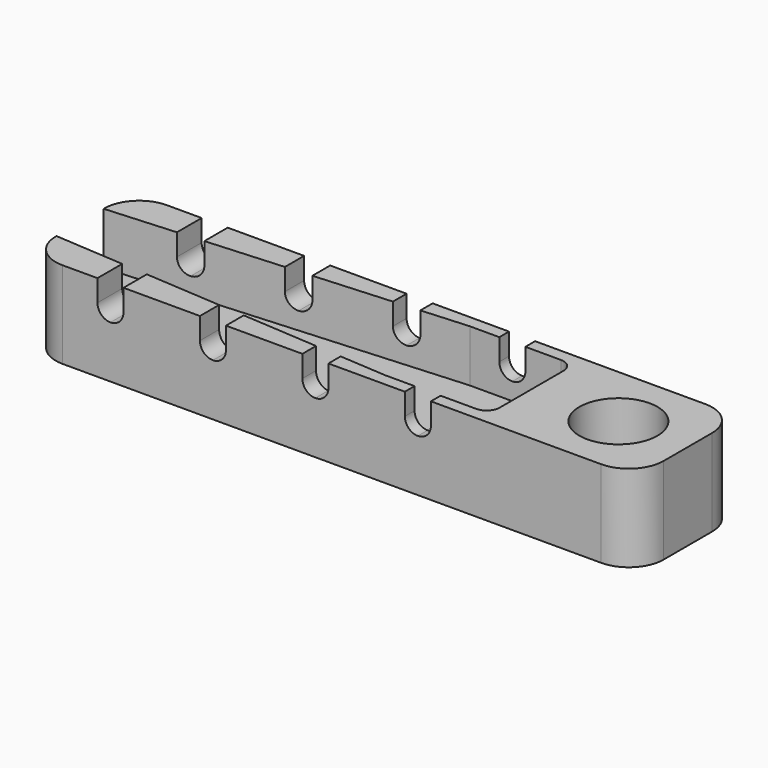
from build123d import *

# Parameters (mm, degrees)
F0_W     = 1.5
F0_H     = 0.7
F0_R     = 2.25
F0_H_2   = 6.1
F0_W_2   = 2.8
F1_DEPTH = 5
F2_DEPTH = 3
F3_DEPTH = 2
F4_R     = 0.74999
F5_R     = 2


# Not quite as in the source:
# - a fillet or chamfer is up to 0.001 mm smaller than in the source, because OpenCascade refuses the exact size


with BuildPart() as f1:
    # F0 (on Top) → F1 (new body)
    with BuildSketch(Plane.XY):
        Polygon((-18.8879279066, 3.75), (-22.8879279066, 3.75), (-22.8879279066, 1.7), (-18.8879279066, 1.97), align=None)
        Polygon((-17.3879279066, 3.75), (-18.8879279066, 3.75), (-18.8879279066, 1.97), (-17.3879279066, 2.07125), align=None)
        Polygon((-18.8879279066, 1.97), (-22.8879279066, 1.7), (-22.8879279066, -1.7), (-18.8879279066, -1.97), align=None)
        Polygon((-12.9879279066, 3.75), (-17.3879279066, 3.75), (-17.3879279066, 2.07125), (-12.9879279066, 2.36825), align=None)
        Polygon((-18.8879279066, -1.97), (-22.8879279066, -1.7), (-22.8879279066, -3.75), (-18.8879279066, -3.75), align=None)
        Polygon((-11.4879279066, 3.75), (-12.9879279066, 3.75), (-12.9879279066, 2.36825), (-11.4879279066, 2.4695), align=None)
        Polygon((-17.3879279066, -2.07125), (-18.8879279066, -1.97), (-18.8879279066, -3.75), (-17.3879279066, -3.75), align=None)
        Polygon((-7.0879279066, 3.75), (-11.4879279066, 3.75), (-11.4879279066, 2.4695), (-7.0879279066, 2.7665), align=None)
        Polygon((-12.9879279066, -2.36825), (-17.3879279066, -2.07125), (-17.3879279066, -3.75), (-12.9879279066, -3.75), align=None)
        Polygon((-5.5879279066, 3.75), (-7.0879279066, 3.75), (-7.0879279066, 2.7665), (-5.5879279066, 2.86775), align=None)
        Polygon((-11.4879279066, -2.4695), (-12.9879279066, -2.36825), (-12.9879279066, -3.75), (-11.4879279066, -3.75), align=None)
        Polygon((-1.1879279066, 3.75), (-5.5879279066, 3.75), (-5.5879279066, 2.86775), (-2.8879279066, 3.05), (-1.1879279066, 3.05), align=None)
        Polygon((-7.0879279066, -2.7665), (-11.4879279066, -2.4695), (-11.4879279066, -3.75), (-7.0879279066, -3.75), align=None)
        with Locations((-0.4379279066, 3.4)):
            Rectangle(F0_W, F0_H)
        Polygon((-5.5879279066, -2.86775), (-7.0879279066, -2.7665), (-7.0879279066, -3.75), (-5.5879279066, -3.75), align=None)
        Polygon((12.1120720934, 3.75), (0.3120720934, 3.75), (0.3120720934, 3.05), (3.1120720934, 3.05), (3.1120720934, -3.05), (0.3120720934, -3.05), (0.3120720934, -3.75), (12.1120720934, -3.75), align=None)
        with Locations((8.1120720934, 0)):
            Circle(F0_R, mode=Mode.SUBTRACT)
        Polygon((-2.8879279066, -3.05), (-5.5879279066, -2.86775), (-5.5879279066, -3.75), (-1.1879279066, -3.75), (-1.1879279066, -3.05), align=None)
        with Locations((-0.4379279066, -3.4)):
            Rectangle(F0_W, F0_H)
        with Locations((-0.4379279066, 0)):
            Rectangle(F0_W, F0_H_2)
        Polygon((-5.5879279066, 2.86775), (-7.0879279066, 2.7665), (-7.0879279066, -2.7665), (-5.5879279066, -2.86775), align=None)
        Polygon((-17.3879279066, 2.07125), (-18.8879279066, 1.97), (-18.8879279066, -1.97), (-17.3879279066, -2.07125), align=None)
        Polygon((-12.9879279066, 2.36825), (-17.3879279066, 2.07125), (-17.3879279066, -2.07125), (-12.9879279066, -2.36825), align=None)
        Polygon((-7.0879279066, 2.7665), (-11.4879279066, 2.4695), (-11.4879279066, -2.4695), (-7.0879279066, -2.7665), align=None)
        Polygon((-11.4879279066, 2.4695), (-12.9879279066, 2.36825), (-12.9879279066, -2.36825), (-11.4879279066, -2.4695), align=None)
        Polygon((-2.8879279066, 3.05), (-5.5879279066, 2.86775), (-5.5879279066, -2.86775), (-2.8879279066, -3.05), (-1.1879279066, -3.05), (-1.1879279066, 3.05), align=None)
        with Locations((1.7120720934, 0)):
            Rectangle(F0_W_2, F0_H_2)
    extrude(amount=-F1_DEPTH)

    # F0 (on Top) → F2 (cut)
    with BuildSketch(Plane.XY):
        Polygon((-18.8879279066, 1.97), (-22.8879279066, 1.7), (-22.8879279066, -1.7), (-18.8879279066, -1.97), align=None)
        Polygon((-17.3879279066, 2.07125), (-18.8879279066, 1.97), (-18.8879279066, -1.97), (-17.3879279066, -2.07125), align=None)
        Polygon((-12.9879279066, 2.36825), (-17.3879279066, 2.07125), (-17.3879279066, -2.07125), (-12.9879279066, -2.36825), align=None)
        Polygon((-11.4879279066, 2.4695), (-12.9879279066, 2.36825), (-12.9879279066, -2.36825), (-11.4879279066, -2.4695), align=None)
        Polygon((-7.0879279066, 2.7665), (-11.4879279066, 2.4695), (-11.4879279066, -2.4695), (-7.0879279066, -2.7665), align=None)
        Polygon((-5.5879279066, 2.86775), (-7.0879279066, 2.7665), (-7.0879279066, -2.7665), (-5.5879279066, -2.86775), align=None)
        Polygon((-2.8879279066, 3.05), (-5.5879279066, 2.86775), (-5.5879279066, -2.86775), (-2.8879279066, -3.05), (-1.1879279066, -3.05), (-1.1879279066, 3.05), align=None)
        with Locations((-0.4379279066, 0)):
            Rectangle(F0_W, F0_H_2)
        with Locations((1.7120720934, 0)):
            Rectangle(F0_W_2, F0_H_2)
    extrude(amount=-F2_DEPTH, mode=Mode.SUBTRACT)

    # F0 (on Top) → F3 (cut)
    with BuildSketch(Plane.XY):
        Polygon((-17.3879279066, 3.75), (-18.8879279066, 3.75), (-18.8879279066, 1.97), (-17.3879279066, 2.07125), align=None)
        Polygon((-11.4879279066, 3.75), (-12.9879279066, 3.75), (-12.9879279066, 2.36825), (-11.4879279066, 2.4695), align=None)
        Polygon((-5.5879279066, 3.75), (-7.0879279066, 3.75), (-7.0879279066, 2.7665), (-5.5879279066, 2.86775), align=None)
        with Locations((-0.4379279066, -3.4)):
            Rectangle(F0_W, F0_H)
        Polygon((-17.3879279066, -2.07125), (-18.8879279066, -1.97), (-18.8879279066, -3.75), (-17.3879279066, -3.75), align=None)
        Polygon((-11.4879279066, -2.4695), (-12.9879279066, -2.36825), (-12.9879279066, -3.75), (-11.4879279066, -3.75), align=None)
        Polygon((-5.5879279066, -2.86775), (-7.0879279066, -2.7665), (-7.0879279066, -3.75), (-5.5879279066, -3.75), align=None)
        with Locations((-0.4379279066, 3.4)):
            Rectangle(F0_W, F0_H)
    extrude(amount=-F3_DEPTH, mode=Mode.SUBTRACT)

    # F4 (radius 0.75 in the source; OpenCascade refuses exactly that, so slightly less here)
    f4_edges = [f1.edges().sort_by_distance(p)[0] for p in [
        (-17.387928, -2.910625, -2),
        (-11.487928, -3.10975, -2),
        (-5.587928, -3.308875, -2),
        (0.312072, -3.4, -2),
        (-18.887928, -2.86, -2),
        (-12.987928, -3.059125, -2),
        (-7.087928, -3.25825, -2),
        (-1.187928, -3.4, -2),
        (-18.887928, 2.86, -2),
        (-12.987928, 3.059125, -2),
        (-7.087928, 3.25825, -2),
        (-1.187928, 3.4, -2),
        (-17.387928, 2.910625, -2),
        (-11.487928, 3.10975, -2),
        (-5.587928, 3.308875, -2),
        (0.312072, 3.4, -2),
        (3.112072, 3.05, -1.5),
        (3.112072, -3.05, -1.5),
    ]]
    fillet(f4_edges, radius=F4_R)

    # F5
    f5_edges = [f1.edges().sort_by_distance(p)[0] for p in [
        (-22.887928, -3.75, -2.5),
        (-22.887928, 3.75, -2.5),
        (12.112072, -3.75, -2.5),
        (12.112072, 3.75, -2.5),
    ]]
    fillet(f5_edges, radius=F5_R)


solid = f1.part
